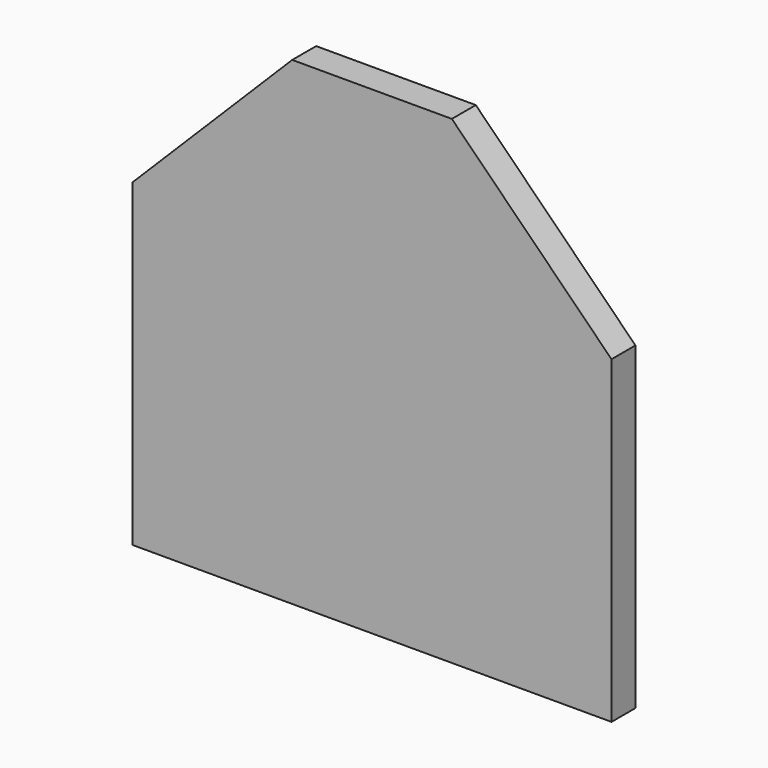
from build123d import *

# Parameters (mm, degrees)
F1_DEPTH = 9.525


# Not quite as in the source:
# - a length typed as a fraction of an inch, garbled in the dataset ("3 / 203.2 mm" for 3/8 in), is restored


with BuildPart() as f1:
    # F0 (on Front) → F1 (new body)
    with BuildSketch(Plane.XZ):
        Polygon((76.2, 25.4), (25.4, 76.2), (-25.4, 76.2), (-76.2, 25.4), (-76.2, -76.2), (76.2, -76.2), align=None)
    extrude(amount=F1_DEPTH)


solid = f1.part
